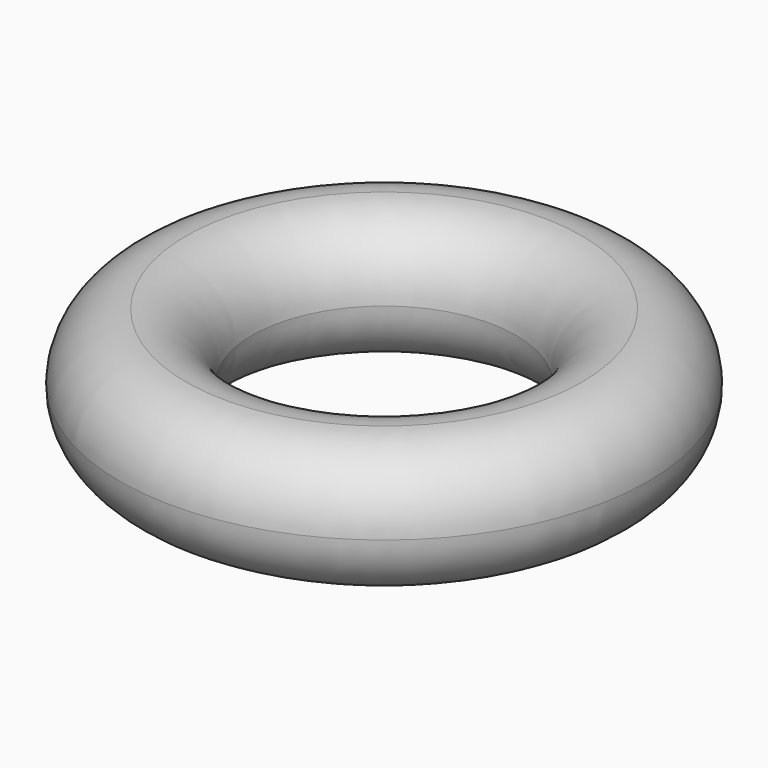
from build123d import *

# Parameters (mm, degrees)
F0_W = 12.7
F0_H = 12.7
F2_R = 6.34999


# Not quite as in the source:
# - a fillet or chamfer is up to 0.001 mm smaller than in the source, because OpenCascade refuses the exact size


with BuildPart() as f1:
    # F0 (on Front) → F1 (revolve)
    with BuildSketch(Plane.XZ):
        with Locations((19.05, 6.35)):
            Rectangle(F0_W, F0_H)
    revolve(axis=Axis((0, 0, 6.35), (0, 0, 1)))

    # F2 (radius 6.35 in the source; OpenCascade refuses exactly that, so slightly less here)
    f2_edges = [f1.edges().sort_by_distance(p)[0] for p in [
        (-25.4, 0, 12.7),
        (-12.7, 0, 12.7),
        (-12.7, 0, 0),
        (-25.4, 0, 0),
    ]]
    fillet(f2_edges, radius=F2_R)


solid = f1.part
